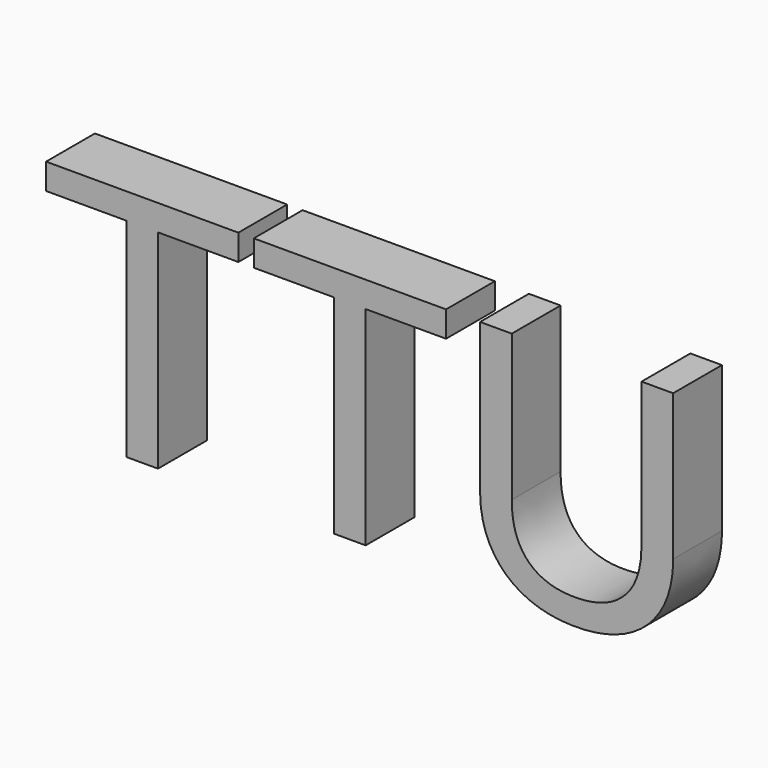
from build123d import *

# Parameters (mm, degrees)
F0_TEXT_SIZE = 11.1464954292
F1_DEPTH     = 2


# Not quite as in the source:
# - Text() gives the source's letters only with a copy of the font that has no kerning and outlines rounded to 1/6400 em; it was checked with that copy


with BuildPart() as f1:
    # F0 (on Front) → F1 (new body)
    with BuildSketch(Plane.XZ):
        with Locations((-6.3953031786, 29.970144853)):
            Text('TTU', F0_TEXT_SIZE, font='Arimo', text_align=(TextAlign.LEFT, TextAlign.BOTTOM))
    extrude(amount=-F1_DEPTH)


solid = f1.part
